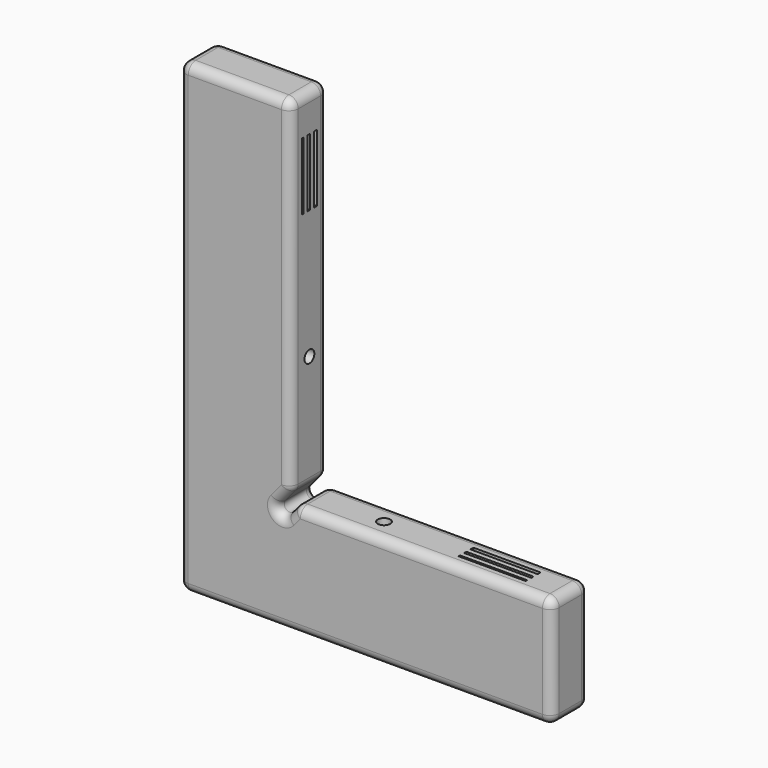
from build123d import *

# Parameters (mm, degrees)
F1_DEPTH     = 25
F2_R         = 5
F3_T1_DEPTH  = 15
F3_S5_W      = 5
F3_S5_H      = 5
F3_T6_DEPTH  = 5
F3_S11_W     = 5
F3_S11_H     = 5
F3_T12_DEPTH = 5
F4_W         = 36
F4_H         = 1
F4_H_2       = 1.5
F4_H_3       = 2
F5_DEPTH     = 64.1
F7_D         = 6.6
F8_W         = 2
F8_H         = 36
F8_W_2       = 1
F8_W_3       = 1.5
F9_DEPTH     = 69
F11_D        = 6.6


# Not quite as in the source:
# - a fillet or chamfer that OpenCascade refuses, or shapes differently, is made with other operations: its cross-section is extruded or revolved along the edge and cut away or added


with BuildPart() as f1:
    # F0 (on Front) → F1 (new body)
    with BuildSketch(Plane.XZ):
        with BuildLine():
            Line((-200, 0), (0, 0))
            Line((0, 0), (0, 60))
            Line((0, 60), (-137.2273796073, 60))
            Line((-137.2273796073, 60), (-142.2018666706, 54.0716371709))
            ThreePointArc((-142.2018666706, 54.0716371709), (-146.4283628291, 53.7018666706), (-146.7981333294, 57.9283628291))
            Line((-146.7981333294, 57.9283628291), (-140, 66.0300626473))
            Line((-140, 66.0300626473), (-140, 250))
            Line((-140, 250), (-200, 250))
            Line((-200, 250), (-200, 0))
        make_face()
    extrude(amount=F1_DEPTH)

    # F2
    f2_edges = [f1.edges().sort_by_distance(p)[0] for p in [
        (-200, -25, 125),
        (-100, -25, 0),
        (0, -25, 30),
        (-68.61369, -25, 60),
        (-139.714623, -25, 57.035819),
        (-146.428363, -25, 53.701867),
        (-143.399067, -25, 61.979213),
        (-140, -25, 158.015031),
        (-170, -25, 250),
        (-100, 0, 0),
        (-200, -12.5, 0),
        (-200, 0, 125),
        (0, 0, 30),
        (-68.61369, 0, 60),
        (-139.714623, 0, 57.035819),
        (-146.428363, 0, 53.701867),
        (-143.399067, 0, 61.979213),
        (-140, 0, 158.015031),
        (-170, 0, 250),
        (0, -12.5, 0),
        (0, -12.5, 60),
        (-137.22738, -12.5, 60),
        (-140, -12.5, 66.030063),
        (-140, -12.5, 250),
    ]]
    fillet(f2_edges, radius=F2_R)

    # F3: fillet of radius 5 on 1 edges, made by hand

    # F3_s2 → F3_t1 (cut)
    with BuildSketch(Plane.XZ.offset(5)):
        with BuildLine():
            ThreePointArc((-200, 245), (-198.5355339059, 248.5355339059), (-195, 250))
            Line((-195, 250), (-200, 250))
            Line((-200, 250), (-200, 245))
        make_face()
    extrude(amount=F3_T1_DEPTH, mode=Mode.SUBTRACT)


with BuildPart() as f3_tool4:
    # F3_s5 → F3_t6 (new body)
    with BuildSketch(Plane.YZ.offset(-195)):
        with Locations((-2.5, 247.5)):
            Rectangle(F3_S5_W, F3_S5_H)
    extrude(amount=-F3_T6_DEPTH)

    # F3_s7 → F3_t8 (revolve, cut)
    with BuildSketch(Plane(origin=(-195, -5, 245), x_dir=(0, -0.7071067812, -0.7071067812), z_dir=(0, 0.7071067812, -0.7071067812))):
        with BuildLine():
            ThreePointArc((0, -5), (5, 0), (0, 5))
            Line((0, 5), (0, -5))
        make_face()
    revolve(axis=Axis((-195, -5, 245), (-1, 0, 0)), mode=Mode.SUBTRACT)


with BuildPart() as f1_1:
    add(f1.part)

    # F3_t3: cut F3_tool4
    add(f3_tool4.part, mode=Mode.SUBTRACT)


with BuildPart() as f3_tool10:
    # F3_s11 → F3_t12 (new body)
    with BuildSketch(Plane.YZ.offset(-195)):
        with Locations((-22.5, 247.5)):
            Rectangle(F3_S11_W, F3_S11_H)
    extrude(amount=-F3_T12_DEPTH)

    # F3_s13 → F3_t14 (revolve, cut)
    with BuildSketch(Plane(origin=(-195, -20, 245), x_dir=(0, 0.7071067812, -0.7071067812), z_dir=(0, 0.7071067812, 0.7071067812))):
        with BuildLine():
            ThreePointArc((0, -5), (5, 0), (0, 5))
            Line((0, 5), (0, -5))
        make_face()
    revolve(axis=Axis((-195, -20, 245), (-1, 0, 0)), mode=Mode.SUBTRACT)


with BuildPart() as f1_2:
    add(f1_1.part)

    # F3_t9: cut F3_tool10
    add(f3_tool10.part, mode=Mode.SUBTRACT)

    # F4 (on face) → F5 (cut)
    with BuildSketch(Plane(origin=(0, 0, 0), x_dir=(1, 0, 0), z_dir=(0, 0, -1))):
        with Locations((-38, 17)):
            Rectangle(F4_W, F4_H)
        with Locations((-38, 13)):
            Rectangle(F4_W, F4_H_2)
        with Locations((-38, 8.5)):
            Rectangle(F4_W, F4_H_3)
    extrude(amount=-F5_DEPTH, mode=Mode.SUBTRACT)

    # F7 (through all)
    with Locations(Plane(origin=(0, 0, 0), x_dir=(1, 0, 0), z_dir=(0, 0, -1))):
        with Locations((-100, 12.5)):
            Hole(F7_D / 2)

    # F8 (on face) → F9 (cut)
    with BuildSketch(Plane(origin=(-200, 0, 0), x_dir=(0, -1, 0), z_dir=(-1, 0, 0))):
        with Locations((8.5, 212)):
            Rectangle(F8_W, F8_H)
        with Locations((17, 212)):
            Rectangle(F8_W_2, F8_H)
        with Locations((13, 212)):
            Rectangle(F8_W_3, F8_H)
    extrude(amount=-F9_DEPTH, mode=Mode.SUBTRACT)

    # F11 (through all)
    with Locations(Plane(origin=(-200, 0, 0), x_dir=(0, -1, 0), z_dir=(-1, 0, 0))):
        with Locations((12.5, 125)):
            Hole(F11_D / 2)


solid = f1_2.part
